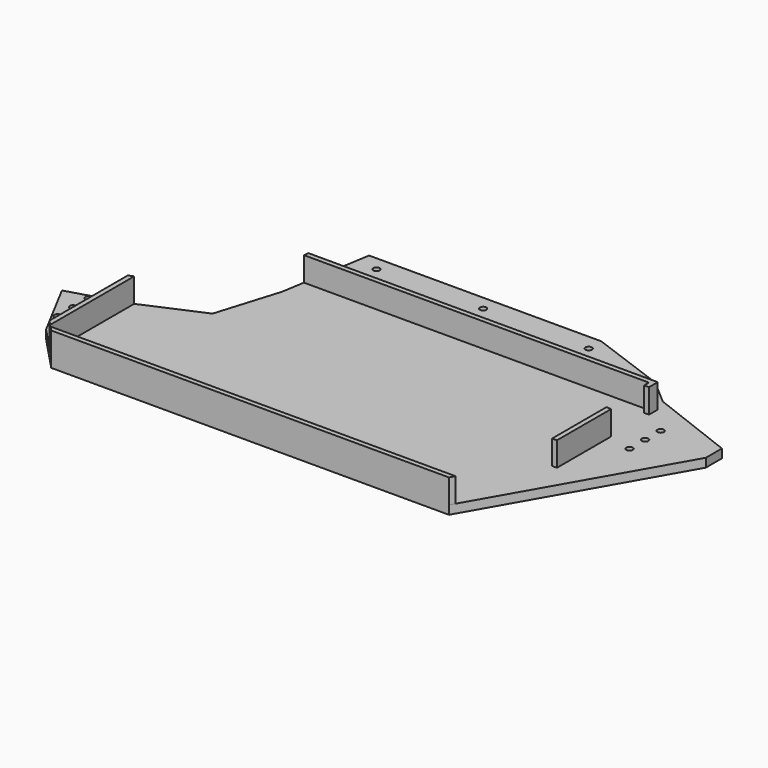
from build123d import *

# Parameters (mm, degrees)
F1_DEPTH      = 2.286
F2_W          = 1.27
F2_H          = 17.78
F3_DEPTH      = 6.35
F3_DEPTH_BACK = 2.286
F4_D          = 1.6933333333


# Not quite as in the source:
# - a feature names something its author has since deleted; it is built from what else it names


with BuildPart() as f1:
    # F0 (on Top) → F1 (new body)
    with BuildSketch(Plane.XY):
        Polygon((-39.7502322496, -19.8751161248), (-31.0001806734, -29.1251689516), (73.3058652154, -29.1251689516), (101.3186621261, 20.063493978), (101.3186621261, 25.3395497125), (78.8771229202, 34.0285638846), (72.3271246897, 39.6729167182), (52.3297434038, 47.023841916), (50.4247434038, 47.023841916), (21.8864718038, 47.023841916), (19.9814718038, 47.023841916), (-8.5567997962, 47.023841916), (-12.4402794499, 23.3751358177), (-17.5001015898, 6.8750406358), (-33.2501941145, 0), (-48.0002794499, -4.3750257881), align=None)
    extrude(amount=F1_DEPTH)

    # F2 (on face) → F3 (join, two sides)
    with BuildSketch(Plane.XY.offset(2.286)) as f3_sk:
        with Locations((79.6558652154, 6.4348310484)):
            Rectangle(F2_W, F2_H)
        Polygon((-32.2015322451, -27.8551689516), (-31.0001806734, -29.1251689516), (73.3058652154, -29.1251689516), (74.0291264296, -27.8551689516), align=None)
        Polygon((80.2908652154, 30.5648310484), (-11.2596214034, 30.5648310484), (-11.4681748498, 29.2948310484), (79.0208652154, 29.2948310484), (79.0208652154, 27.7073310484), (80.2908652154, 27.7073310484), align=None)
        Polygon((-34.0091347846, -0.2251095453), (-34.0091347846, -25.944275189), (-32.7391347846, -27.2868463713), (-32.7391347846, 0.2230814616), (-33.2501941145, 0), align=None)
    extrude(amount=F3_DEPTH)
    extrude(f3_sk.sketch, amount=-F3_DEPTH_BACK)

    # F4 (through all)
    with Locations(Plane.XY.offset(2.286)):
        with Locations((-41.6291347846, -13.7730257881), (-41.6291347846, -8.6930257881), (-41.6291347846, -3.6130257881), (-3.5502565962, 43.2212361431), (-3.5502565962, 38.1412361431), (-3.5502565962, 33.0612361431), (24.3897434038, 43.2212361431), (24.3897434038, 38.1412361431), (24.3897434038, 33.0612361431), (52.3297434038, 42.9037361431), (52.3297434038, 37.8237361431), (52.3297434038, 32.7437361431), (86.6408652154, 23.6032530031), (86.6408652154, 18.5232530031), (86.6408652154, 13.4432530031)):
            Hole(F4_D / 2)


solid = f1.part
